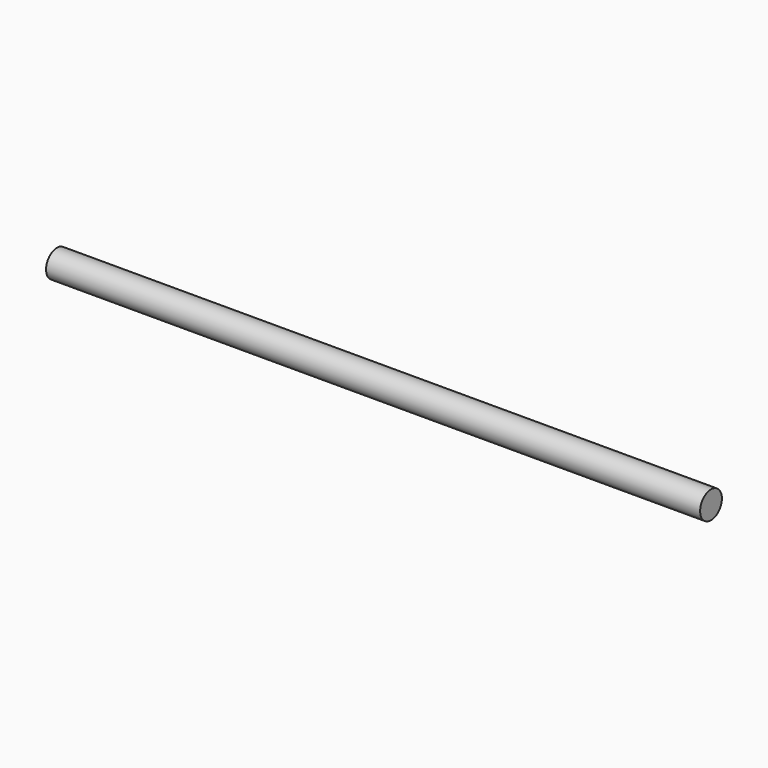
from build123d import *

# Parameters (mm, degrees)
F1_R     = 6.35
F2_DEPTH = 304.8


# Not quite as in the source:
# - a variable given as a bare number and used for a length is read in inches; the dataset says mm whatever the document's units were


with BuildPart() as f2:
    # F1 (on Right) → F2 (new body)
    with BuildSketch(Plane.YZ):
        Circle(F1_R)
    extrude(amount=F2_DEPTH)


solid = f2.part
